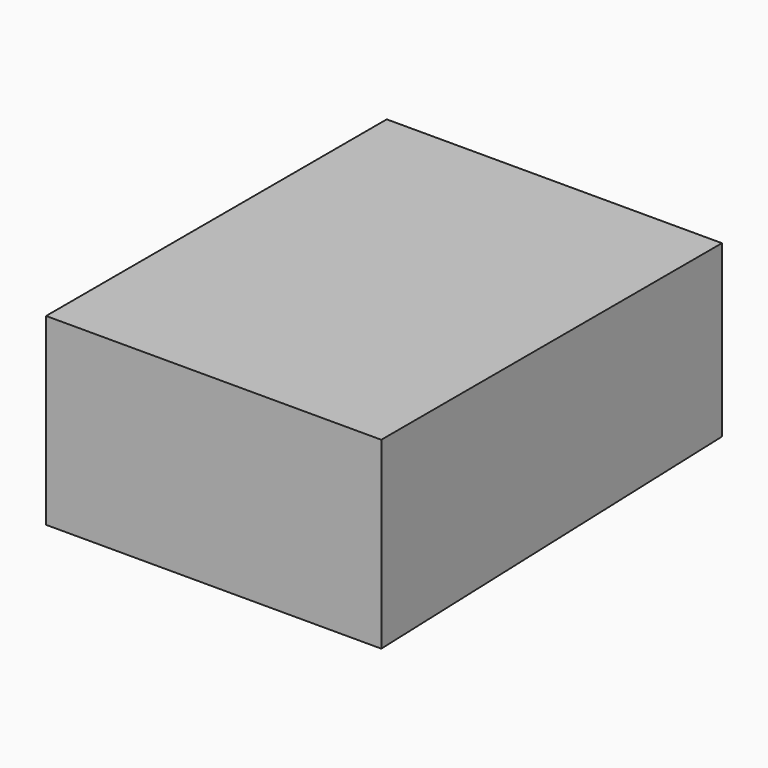
from build123d import *

# Parameters (mm, degrees)
F0_W     = 3700
F0_H     = 4700
F1_DEPTH = 1520
F3_DEPTH = 3700


# Not quite as in the source:
# - the program builds the solid bodies; features that only make, move or delete a surface that nothing else refers to are left out


with BuildPart() as f1:
    # F0 (on Top) → F1 (new body)
    with BuildSketch(Plane.XY):
        with Locations((1850, 2350)):
            Rectangle(F0_W, F0_H)
    extrude(amount=F1_DEPTH)

    # F2 (on face) → F3 (join)
    with BuildSketch(Plane.YZ.offset(3700)):
        Polygon((4700, 0), (0, 0), (0, -510), (4700, -360), align=None)
    extrude(amount=-F3_DEPTH)


solid = f1.part
